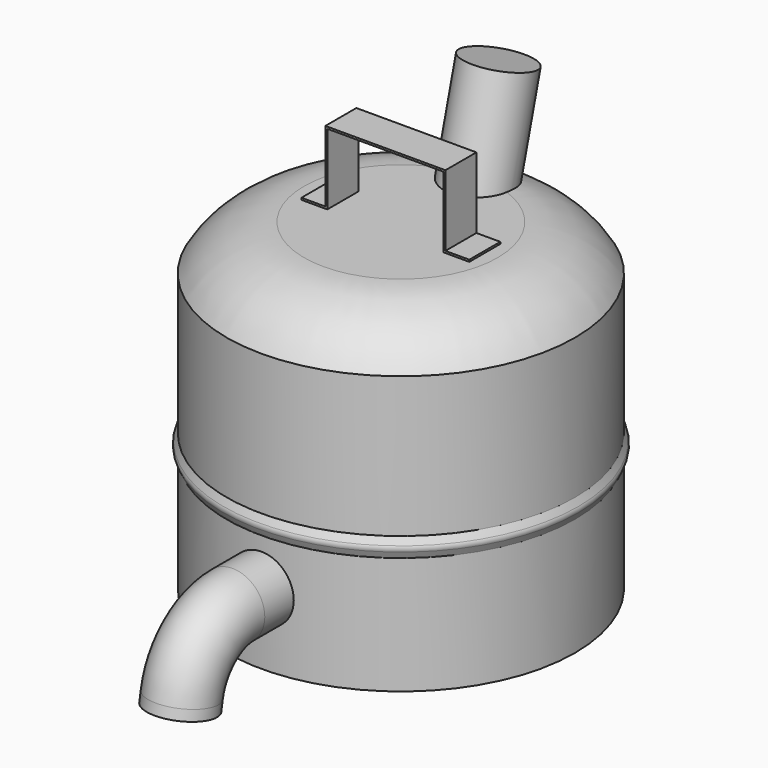
from build123d import *

# Parameters (mm, degrees)
F0_R      = 135
F1_DEPTH  = 215
F5_DEPTH  = 15
F10_R     = 26
F11_DEPTH = 75
F13_R     = 25


with BuildPart() as f1:
    # F0 (on Top) → F1 (new body)
    with BuildSketch(Plane.XY):
        Circle(F0_R)
    extrude(amount=F1_DEPTH)

    # F2 (on Right) → F3 (revolve)
    with BuildSketch(Plane.YZ):
        with BuildLine():
            ThreePointArc((-75, 250), (-109.6475910005, 240.467298858), (-135, 215))
            Line((-135, 215), (0, 215))
            Line((0, 215), (0, 250))
            Line((0, 250), (-75, 250))
        make_face()
    revolve(axis=Axis((0, 0, 232.5), (0, 0, 1)))

    # F10 (on face) → F11 (join, symmetric)
    with BuildSketch(Plane(origin=(0, 67.5240473581, 252.0031754731), x_dir=(1, 0, 0), z_dir=(0, 0.2588190451, 0.9659258263))):
        with Locations((0, 7.739675696)):
            Circle(F10_R)
    extrude(amount=F11_DEPTH, both=True)

    # F16 (on Front) → F17 (revolve)
    with BuildSketch(Plane.XZ):
        with BuildLine():
            Line((137.5252101931, 100.6266106152), (135, 106))
            Line((135, 106), (135, 91))
            Line((135, 91), (137.5252101931, 96.3733893848))
            ThreePointArc((137.5252101931, 96.3733893848), (138, 98.5), (137.5252101931, 100.6266106152))
        make_face()
    revolve(axis=Axis((0, 0, 0), (0, 0, 1)))


with BuildPart() as f5:
    # F4 (on Front) → F5 (new body, symmetric)
    with BuildSketch(Plane.XZ):
        Polygon((-65, 251.5), (-65, 250), (-45, 250), (-45, 305), (0, 305), (0, 306.5), (-46.5, 306.5), (-46.5, 251.5), align=None)
    extrude(amount=F5_DEPTH, both=True)

    # F6: F5 across plane


with BuildPart() as f5_1:
    add(f5.part)
    add(f5.part.mirror(Plane.YZ))


with BuildPart() as f15:
    # F15: sweep along a path in F14
    with BuildLine(Plane.YZ) as f15_path:
        Line((-135, 55), (-163.0450184411, 55))
        ThreePointArc((-163.0450184411, 55), (-195.1843989255, 43.3022221559), (-212.2854060917, 13.6824088833))
        Line((-212.2854060917, 13.6824088833), (-213.6824088833, 5.7596123494))
    # F13 (on offset) → F15 (sweep)
    with BuildSketch(Plane.XZ.offset(135)):
        with Locations((0, 55)):
            Circle(F13_R)
    sweep(path=f15_path.line)


solid = Compound([f1.part, f5_1.part, f15.part])
